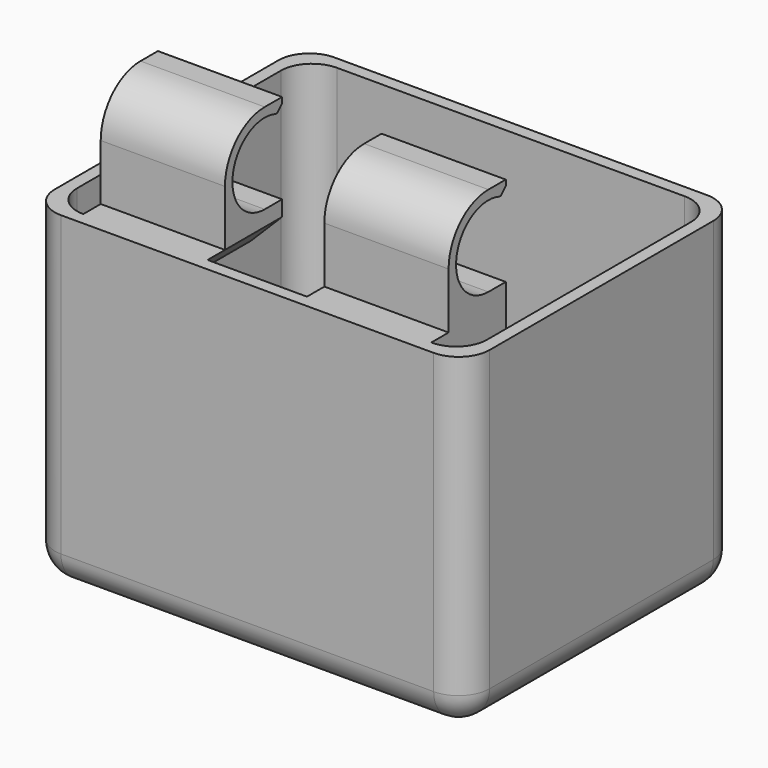
from build123d import *

# Parameters (mm, degrees)
F0_W         = 70
F0_H         = 55
F0_W_2       = 49.5
F0_H_2       = 29.3
F1_DEPTH     = 3
F2_R         = 1.5
F2_W         = 49.5
F2_H         = 29.3
F3_DEPTH     = 10
F2_W_2       = 70
F2_H_2       = 55
F2_W_3       = 66
F2_H_3       = 51
F4_DEPTH     = 50
F5_T1_DEPTH  = 45
F5_T3_DEPTH  = 41
F5_S7_W      = 5.1
F5_S7_H      = 5.1
F5_T8_DEPTH  = 5.1
F5_S13_W     = 5.1
F5_S13_H     = 5.1
F5_T14_DEPTH = 5.1
F5_S19_W     = 5.1
F5_S19_H     = 5.1
F5_T20_DEPTH = 5.1
F5_S25_W     = 5.1
F5_S25_H     = 5.1
F5_T26_DEPTH = 5.1
F5_T32_DEPTH = 56
F5_S33_R     = 4.5
F5_T34_DEPTH = 30
F5_T38_DEPTH = 56
F5_S39_R     = 4.5
F5_T40_DEPTH = 30
F5_T41_DEPTH = 45
F5_T43_DEPTH = 60.5
F5_T45_DEPTH = 60
F5_S49_W     = 5.1
F5_S49_H     = 5.1
F5_T50_DEPTH = 5.1
F5_S55_W     = 5.1
F5_S55_H     = 5.1
F5_T56_DEPTH = 5.1
F5_S61_W     = 5.1
F5_S61_H     = 5.1
F5_T62_DEPTH = 5.1
F5_S67_W     = 5.1
F5_S67_H     = 5.1
F5_T68_DEPTH = 5.1
F6_W         = 20
F6_H         = 15
F7_DEPTH     = 2
F9_DEPTH     = 56
F10_W        = 16
F10_H        = 9
F10_H_2      = 13.2445012331
F11_DEPTH    = 25
F12_DEPTH    = 3
F13_SIZE     = 4.99999
F14_SIZE     = 1


# Not quite as in the source:
# - a fillet or chamfer that OpenCascade refuses, or shapes differently, is made with other operations: its cross-section is extruded or revolved along the edge and cut away or added
# - a fillet or chamfer is up to 0.001 mm smaller than in the source, because OpenCascade refuses the exact size


with BuildPart() as f1:
    # F0 (on Top) → F1 (new body)
    with BuildSketch(Plane.XY):
        Rectangle(F0_W, F0_H)
        Rectangle(F0_W_2, F0_H_2, mode=Mode.SUBTRACT)
    extrude(amount=F1_DEPTH)

    # F2 (on face) → F3 (join)
    with BuildSketch(Plane.XY.offset(3)):
        with BuildLine():
            Line((-3.2619012861, 16.65), (-26.75, 16.65))
            Line((-26.75, 16.65), (-26.75, -16.65))
            Line((-26.75, -16.65), (-3.2619012861, -16.65))
            ThreePointArc((-3.2619012861, -16.65), (0, -24.25), (3.2619012861, -16.65))
            Line((3.2619012861, -16.65), (26.75, -16.65))
            Line((26.75, -16.65), (26.75, 16.65))
            Line((26.75, 16.65), (3.2619012861, 16.65))
            ThreePointArc((3.2619012861, 16.65), (0, 24.25), (-3.2619012861, 16.65))
        make_face()
        with Locations((0, -19.75)):
            Circle(F2_R, mode=Mode.SUBTRACT)
        Rectangle(F2_W, F2_H, mode=Mode.SUBTRACT)
        with Locations((0, 19.75)):
            Circle(F2_R, mode=Mode.SUBTRACT)
    extrude(amount=F3_DEPTH)

    # F2 (on face) → F4 (join)
    with BuildSketch(Plane.XY.offset(3)):
        Rectangle(F2_W_2, F2_H_2)
        Rectangle(F2_W_3, F2_H_3, mode=Mode.SUBTRACT)
    extrude(amount=F4_DEPTH)

    # F5: fillet of radius 5 on 16 edges, made by hand

    # F5_s2 → F5_t1 (join)
    with BuildSketch(Plane.XY.offset(8)):
        with BuildLine():
            ThreePointArc((-33, 20.5), (-31.5355339059, 24.0355339059), (-28, 25.5))
            Line((-28, 25.5), (-33, 25.5))
            Line((-33, 25.5), (-33, 20.5))
        make_face()
        with BuildLine():
            ThreePointArc((33, 20.5), (31.5355339059, 24.0355339059), (28, 25.5))
            Line((28, 25.5), (33, 25.5))
            Line((33, 25.5), (33, 20.5))
        make_face()
        with BuildLine():
            ThreePointArc((-33, -20.5), (-31.5355339059, -24.0355339059), (-28, -25.5))
            Line((-28, -25.5), (-33, -25.5))
            Line((-33, -25.5), (-33, -20.5))
        make_face()
        with BuildLine():
            ThreePointArc((28, -25.5), (31.5355339059, -24.0355339059), (33, -20.5))
            Line((33, -20.5), (33, -25.5))
            Line((33, -25.5), (28, -25.5))
        make_face()
    extrude(amount=F5_T1_DEPTH)

    # F5_s4 → F5_t3 (join)
    with BuildSketch(Plane.XZ.offset(-20.5)):
        with BuildLine():
            ThreePointArc((-28, 3), (-31.5355339059, 4.4644660941), (-33, 8))
            Line((-33, 8), (-33, 3))
            Line((-33, 3), (-28, 3))
        make_face()
        with BuildLine():
            ThreePointArc((28, 3), (31.5355339059, 4.4644660941), (33, 8))
            Line((33, 8), (33, 3))
            Line((33, 3), (28, 3))
        make_face()
    extrude(amount=F5_T3_DEPTH)


with BuildPart() as f5_tool6:
    # F5_s7 → F5_t8 (new body)
    with BuildSketch(Plane.XY.offset(8)):
        with Locations((-30.55, 23.05)):
            Rectangle(F5_S7_W, F5_S7_H)
    extrude(amount=-F5_T8_DEPTH)

    # F5_s9 → F5_t10 (revolve, cut)
    with BuildSketch(Plane(origin=(-28, 20.5, 8), x_dir=(0.7071067812, -0.7071067812, 0), z_dir=(0.7071067812, 0.7071067812, 0))):
        with BuildLine():
            ThreePointArc((0, -5), (5, 0), (0, 5))
            Line((0, 5), (0, -5))
        make_face()
    revolve(axis=Axis((-28, 20.5, 8), (0, 0, -1)), mode=Mode.SUBTRACT)


with BuildPart() as f1_1:
    add(f1.part)

    # F5_t5: union F5_tool6
    add(f5_tool6.part)


with BuildPart() as f5_tool12:
    # F5_s13 → F5_t14 (new body)
    with BuildSketch(Plane.XY.offset(8)):
        with Locations((30.55, 23.05)):
            Rectangle(F5_S13_W, F5_S13_H)
    extrude(amount=-F5_T14_DEPTH)

    # F5_s15 → F5_t16 (revolve, cut)
    with BuildSketch(Plane(origin=(28, 20.5, 8), x_dir=(-0.7071067812, -0.7071067812, 0), z_dir=(0.7071067812, -0.7071067812, 0))):
        with BuildLine():
            ThreePointArc((0, -5), (5, 0), (0, 5))
            Line((0, 5), (0, -5))
        make_face()
    revolve(axis=Axis((28, 20.5, 8), (0, 0, -1)), mode=Mode.SUBTRACT)


with BuildPart() as f1_2:
    add(f1_1.part)

    # F5_t11: union F5_tool12
    add(f5_tool12.part)


with BuildPart() as f5_tool18:
    # F5_s19 → F5_t20 (new body)
    with BuildSketch(Plane.XY.offset(8)):
        with Locations((-30.55, -23.05)):
            Rectangle(F5_S19_W, F5_S19_H)
    extrude(amount=-F5_T20_DEPTH)

    # F5_s21 → F5_t22 (revolve, cut)
    with BuildSketch(Plane(origin=(-28, -20.5, 8), x_dir=(0.7071067812, 0.7071067812, 0), z_dir=(-0.7071067812, 0.7071067812, 0))):
        with BuildLine():
            ThreePointArc((0, -5), (5, 0), (0, 5))
            Line((0, 5), (0, -5))
        make_face()
    revolve(axis=Axis((-28, -20.5, 8), (0, 0, -1)), mode=Mode.SUBTRACT)


with BuildPart() as f1_3:
    add(f1_2.part)

    # F5_t17: union F5_tool18
    add(f5_tool18.part)


with BuildPart() as f5_tool24:
    # F5_s25 → F5_t26 (new body)
    with BuildSketch(Plane.XY.offset(8)):
        with Locations((30.55, -23.05)):
            Rectangle(F5_S25_W, F5_S25_H)
    extrude(amount=-F5_T26_DEPTH)

    # F5_s27 → F5_t28 (revolve, cut)
    with BuildSketch(Plane(origin=(28, -20.5, 8), x_dir=(-0.7071067812, 0.7071067812, 0), z_dir=(-0.7071067812, -0.7071067812, 0))):
        with BuildLine():
            ThreePointArc((0, -5), (5, 0), (0, 5))
            Line((0, 5), (0, -5))
        make_face()
    revolve(axis=Axis((28, -20.5, 8), (0, 0, -1)), mode=Mode.SUBTRACT)


with BuildPart() as f1_4:
    add(f1_3.part)

    # F5_t23: union F5_tool24
    add(f5_tool24.part)


with BuildPart() as f5_tool30:
    # F5_s31 → F5_t32 (new body)
    with BuildSketch(Plane.YZ.offset(-28)):
        with BuildLine():
            ThreePointArc((20.5, 3), (24.0355339059, 4.4644660941), (25.5, 8))
            Line((25.5, 8), (25.5, 3))
            Line((25.5, 3), (20.5, 3))
        make_face()
    extrude(amount=F5_T32_DEPTH)

    # F5_s33 → F5_t34 (cut, symmetric)
    with BuildSketch(Plane.XY.offset(5.5)):
        with Locations((0, 19.75)):
            Circle(F5_S33_R)
    extrude(amount=F5_T34_DEPTH, both=True, mode=Mode.SUBTRACT)


with BuildPart() as f1_5:
    add(f1_4.part)

    # F5_t29: union F5_tool30
    add(f5_tool30.part)


with BuildPart() as f5_tool36:
    # F5_s37 → F5_t38 (new body)
    with BuildSketch(Plane.YZ.offset(28)):
        with BuildLine():
            ThreePointArc((-20.5, 3), (-24.0355339059, 4.4644660941), (-25.5, 8))
            Line((-25.5, 8), (-25.5, 3))
            Line((-25.5, 3), (-20.5, 3))
        make_face()
    extrude(amount=-F5_T38_DEPTH)

    # F5_s39 → F5_t40 (cut, symmetric)
    with BuildSketch(Plane.XY.offset(5.5)):
        with Locations((0, -19.75)):
            Circle(F5_S39_R)
    extrude(amount=F5_T40_DEPTH, both=True, mode=Mode.SUBTRACT)


with BuildPart() as f1_6:
    add(f1_5.part)

    # F5_t35: union F5_tool36
    add(f5_tool36.part)

    # F5_s42 → F5_t41 (cut)
    with BuildSketch(Plane.XZ.offset(-22.5)):
        with BuildLine():
            ThreePointArc((-30, 0), (-33.5355339059, 1.4644660941), (-35, 5))
            Line((-35, 5), (-35, 0))
            Line((-35, 0), (-30, 0))
        make_face()
        with BuildLine():
            ThreePointArc((35, 5), (33.5355339059, 1.4644660941), (30, 0))
            Line((30, 0), (35, 0))
            Line((35, 0), (35, 5))
        make_face()
    extrude(amount=F5_T41_DEPTH, mode=Mode.SUBTRACT)

    # F5_s44 → F5_t43 (cut)
    with BuildSketch(Plane.XY.offset(5)):
        with BuildLine():
            ThreePointArc((-30, 27.5), (-33.5355339059, 26.0355339059), (-35, 22.5))
            Line((-35, 22.5), (-35, 27.5))
            Line((-35, 27.5), (-30, 27.5))
        make_face()
        with BuildLine():
            ThreePointArc((-30, -27.5), (-33.5355339059, -26.0355339059), (-35, -22.5))
            Line((-35, -22.5), (-35, -27.5))
            Line((-35, -27.5), (-30, -27.5))
        make_face()
        with BuildLine():
            ThreePointArc((35, 22.5), (33.5355339059, 26.0355339059), (30, 27.5))
            Line((30, 27.5), (35, 27.5))
            Line((35, 27.5), (35, 22.5))
        make_face()
        with BuildLine():
            ThreePointArc((35, -22.5), (33.5355339059, -26.0355339059), (30, -27.5))
            Line((30, -27.5), (35, -27.5))
            Line((35, -27.5), (35, -22.5))
        make_face()
    extrude(amount=F5_T43_DEPTH, mode=Mode.SUBTRACT)

    # F5_s46 → F5_t45 (cut)
    with BuildSketch(Plane.YZ.offset(-30)):
        with BuildLine():
            ThreePointArc((27.5, 5), (26.0355339059, 1.4644660941), (22.5, 0))
            Line((22.5, 0), (27.5, 0))
            Line((27.5, 0), (27.5, 5))
        make_face()
        with BuildLine():
            ThreePointArc((-27.5, 5), (-26.0355339059, 1.4644660941), (-22.5, 0))
            Line((-22.5, 0), (-27.5, 0))
            Line((-27.5, 0), (-27.5, 5))
        make_face()
    extrude(amount=F5_T45_DEPTH, mode=Mode.SUBTRACT)


with BuildPart() as f5_tool48:
    # F5_s49 → F5_t50 (new body)
    with BuildSketch(Plane.XZ.offset(-22.5)):
        with Locations((-32.55, 2.45)):
            Rectangle(F5_S49_W, F5_S49_H)
    extrude(amount=-F5_T50_DEPTH)

    # F5_s51 → F5_t52 (revolve, cut)
    with BuildSketch(Plane(origin=(-30, 22.5, 5), x_dir=(0.7071067812, 0, 0.7071067812), z_dir=(-0.7071067812, 0, 0.7071067812))):
        with BuildLine():
            ThreePointArc((0, -5), (5, 0), (0, 5))
            Line((0, 5), (0, -5))
        make_face()
    revolve(axis=Axis((-30, 22.5, 5), (0, 1, 0)), mode=Mode.SUBTRACT)


with BuildPart() as f1_7:
    add(f1_6.part)

    # F5_t47: cut F5_tool48
    add(f5_tool48.part, mode=Mode.SUBTRACT)


with BuildPart() as f5_tool54:
    # F5_s55 → F5_t56 (new body)
    with BuildSketch(Plane.XZ.offset(22.5)):
        with Locations((-32.55, 2.45)):
            Rectangle(F5_S55_W, F5_S55_H)
    extrude(amount=F5_T56_DEPTH)

    # F5_s57 → F5_t58 (revolve, cut)
    with BuildSketch(Plane(origin=(-30, -22.5, 5), x_dir=(0.7071067812, 0, 0.7071067812), z_dir=(0.7071067812, 0, -0.7071067812))):
        with BuildLine():
            ThreePointArc((0, -5), (5, 0), (0, 5))
            Line((0, 5), (0, -5))
        make_face()
    revolve(axis=Axis((-30, -22.5, 5), (0, -1, 0)), mode=Mode.SUBTRACT)


with BuildPart() as f1_8:
    add(f1_7.part)

    # F5_t53: cut F5_tool54
    add(f5_tool54.part, mode=Mode.SUBTRACT)


with BuildPart() as f5_tool60:
    # F5_s61 → F5_t62 (new body)
    with BuildSketch(Plane.YZ.offset(30)):
        with Locations((25.05, 2.45)):
            Rectangle(F5_S61_W, F5_S61_H)
    extrude(amount=F5_T62_DEPTH)

    # F5_s63 → F5_t64 (revolve, cut)
    with BuildSketch(Plane(origin=(30, 22.5, 5), x_dir=(0, -0.7071067812, 0.7071067812), z_dir=(0, 0.7071067812, 0.7071067812))):
        with BuildLine():
            ThreePointArc((0, -5), (5, 0), (0, 5))
            Line((0, 5), (0, -5))
        make_face()
    revolve(axis=Axis((30, 22.5, 5), (1, 0, 0)), mode=Mode.SUBTRACT)


with BuildPart() as f1_9:
    add(f1_8.part)

    # F5_t59: cut F5_tool60
    add(f5_tool60.part, mode=Mode.SUBTRACT)


with BuildPart() as f5_tool66:
    # F5_s67 → F5_t68 (new body)
    with BuildSketch(Plane.YZ.offset(30)):
        with Locations((-25.05, 2.45)):
            Rectangle(F5_S67_W, F5_S67_H)
    extrude(amount=F5_T68_DEPTH)

    # F5_s69 → F5_t70 (revolve, cut)
    with BuildSketch(Plane(origin=(30, -22.5, 5), x_dir=(0, 0.7071067812, 0.7071067812), z_dir=(0, 0.7071067812, -0.7071067812))):
        with BuildLine():
            ThreePointArc((0, -5), (5, 0), (0, 5))
            Line((0, 5), (0, -5))
        make_face()
    revolve(axis=Axis((30, -22.5, 5), (1, 0, 0)), mode=Mode.SUBTRACT)


with BuildPart() as f1_10:
    add(f1_9.part)

    # F5_t65: cut F5_tool66
    add(f5_tool66.part, mode=Mode.SUBTRACT)

    # F6 (on face) → F7 (join)
    with BuildSketch(Plane.XY.offset(53)):
        with Locations((18, -18)):
            Rectangle(F6_W, F6_H)
        with Locations((-18, -18)):
            Rectangle(F6_W, F6_H)
    extrude(amount=-F7_DEPTH)

    # F8 (on face) → F9 (join)
    with BuildSketch(Plane.YZ.offset(28)):
        with BuildLine():
            ThreePointArc((-14, 55.5), (-20.4012503946, 63.1287131548), (-11.7768690684, 68.1080020351))
            Line((-11.7768690684, 68.1080020351), (-10.5, 68.1080020351))
            Line((-10.5, 68.1080020351), (-10.5, 70))
            Line((-10.5, 70), (-14, 70))
            ThreePointArc((-14, 70), (-19.6568542495, 67.6568542495), (-22, 62))
            Line((-22, 62), (-22, 53))
            Line((-22, 53), (-10.5, 53))
            Line((-10.5, 53), (-10.5, 55.5))
            Line((-10.5, 55.5), (-14, 55.5))
        make_face()
    extrude(amount=-F9_DEPTH)

    # F10 (on face) → F11 (cut)
    with BuildSketch(Plane.XZ.offset(22)):
        with Locations((0, 57.5)):
            Rectangle(F10_W, F10_H)
        with Locations((0, 68.6222506166)):
            Rectangle(F10_W, F10_H_2)
    extrude(amount=-F11_DEPTH, mode=Mode.SUBTRACT)

    # F12 (add): faces of the model
    f12_faces = [f1_10.faces().sort_by_distance(p)[0] for p in [
        (18, -18, 51),
        (-18, -18, 51),
    ]]
    extrude(f12_faces, amount=F12_DEPTH)

    # F13 (size 5 in the source; OpenCascade refuses exactly that, so slightly less here)
    f13_edges = [f1_10.edges().sort_by_distance(p)[0] for p in [
        (-8, -18, 48),
        (8, -18, 48),
    ]]
    chamfer(f13_edges, length=F13_SIZE)

    # F14
    f14_edges = [f1_10.edges().sort_by_distance(p)[0] for p in [
        (18, -10.5, 68.108002),
        (-18, -10.5, 68.108002),
    ]]
    chamfer(f14_edges, length=F14_SIZE)


solid = f1_10.part
